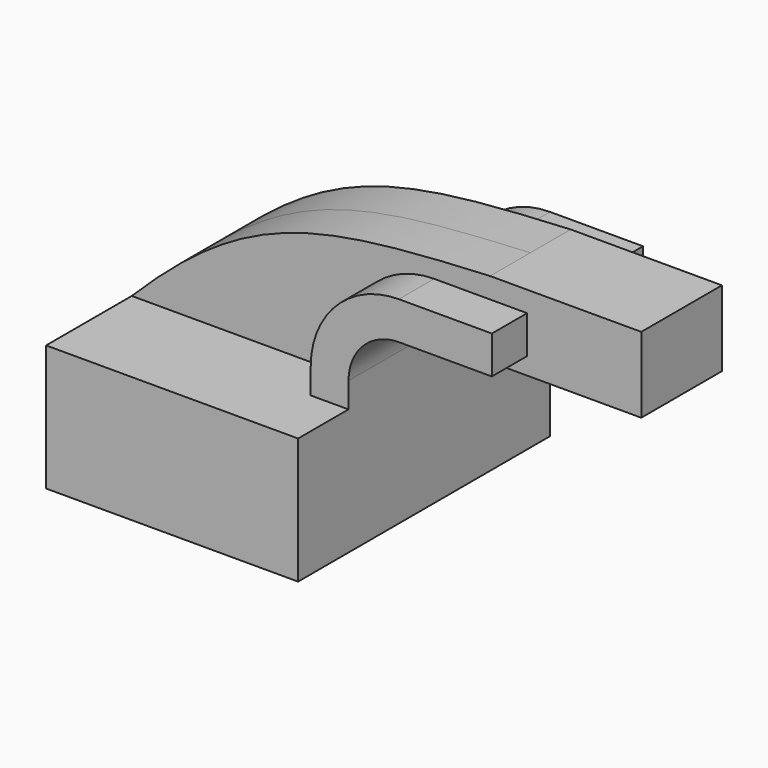
from build123d import *

# Parameters (mm, degrees)
F1_DEPTH = 62.5
F0_W     = 14.7052842798
F0_H     = 15
F2_DEPTH = 37.5
F0_H_2   = 6.8016763031
F0_H_3   = 8.1983236969
F3_DEPTH = 20


with BuildPart() as f1:
    # F0 (on Front) → F1 (new body, symmetric)
    with BuildSketch(Plane.XZ):
        Polygon((-50, 25), (-50, -25), (50, -25), (50, 25), (35, 25), align=None)
    extrude(amount=F1_DEPTH, both=True)

    # F0 (on Front) → F2 (join, symmetric)
    with BuildSketch(Plane.XZ):
        with Locations((99.52410253, 62.5)):
            Rectangle(F0_W, F0_H)
        with BuildLine():
            Line((35, 25), (50, 25))
            Line((50, 25), (50, 35))
            ThreePointArc((50, 35), (55.8578643763, 49.1421356237), (70, 55))
            Line((70, 55), (92.1714603901, 55))
            Line((92.1714603901, 55), (92.1714603901, 70))
            Line((92.1714603901, 70), (70, 70))
            ThreePointArc((70, 70), (45.2512626585, 59.7487373415), (35, 35))
            Line((35, 35), (35, 25))
        make_face()
    extrude(amount=F2_DEPTH, both=True)

    # F0 (on Front) → F3 (join, symmetric)
    with BuildSketch(Plane.XZ):
        with BuildLine():
            add(Edge.make_bspline(
                [(-50, 25), (-4.2251776904, 70.7326084375), (24.2556538433, 74.8012959957), (92.1714603901, 78.1983236969)],
                knots=[0, 0, 0, 0, 151.7985039241, 151.7985039241, 151.7985039241, 151.7985039241], degree=3))
            Line((-50, 25), (35, 25))
            Line((35, 25), (35, 35))
            ThreePointArc((35, 35), (45.2512626585, 59.7487373415), (70, 70))
            Line((70, 70), (92.1714603901, 70))
            Line((92.1714603901, 70), (92.1714603901, 78.1983236969))
        make_face()
        Polygon((106.8767446699, 48.1983236969), (137.2651457787, 48.1983236969), (152.1714603901, 48.1983236969), (152.1714603901, 78.1983236969), (127.8208345175, 78.1983236969), (106.8767446699, 78.1983236969), (106.8767446699, 70), (106.8767446699, 55), align=None)
        with Locations((99.52410253, 51.5991618484)):
            Rectangle(F0_W, F0_H_2)
        with Locations((99.52410253, 74.0991618484)):
            Rectangle(F0_W, F0_H_3)
    extrude(amount=F3_DEPTH, both=True)


solid = f1.part
